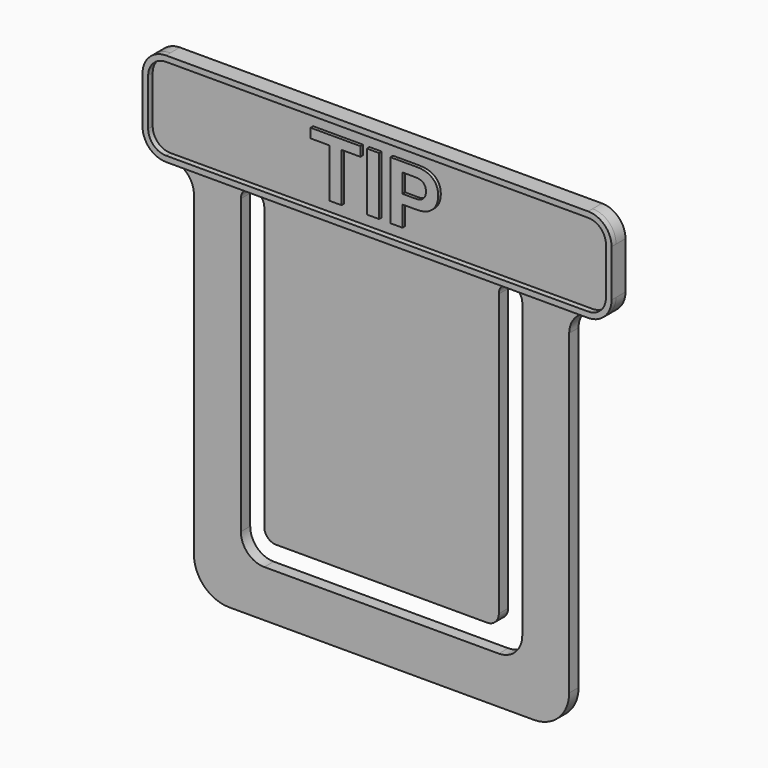
from build123d import *

# Parameters (mm, degrees)
F0_W          = 25.4
F0_H          = 25.4
F1_DEPTH      = 0.79375
F2_R          = 2.38125
F3_W          = 19.05
F3_H          = 22.225
F4_DEPTH      = 4.9276
F6_DEPTH      = 0.79375
F7_R          = 1.58749
F8_R          = 1.5875
F9_W          = 15.875
F9_H          = 20.6375
F10_DEPTH     = 0.79375
F11_R         = 0.79374
F12_R         = 0.79375
F14_DEPTH     = 0.381
F16_DEPTH     = 0.381
F17_TEXT_SIZE = 5.7207213508
F18_DEPTH     = 1.016


# Not quite as in the source:
# - a fillet or chamfer is up to 0.001 mm smaller than in the source, because OpenCascade refuses the exact size
# - ends of sketch curves that miss each other by under 0.0002 mm in the source are joined
# - Text() gives the source's letters only with a copy of the font that has no kerning and outlines rounded to 1/6400 em; it was checked with that copy


with BuildPart() as f1:
    # F0 (on Front) → F1 (new body)
    with BuildSketch(Plane.XZ):
        Rectangle(F0_W, F0_H)
    extrude(amount=F1_DEPTH)

    # F2
    f2_edges = [f1.edges().sort_by_distance(p)[0] for p in [
        (12.7, -0.396875, -12.7),
        (-12.7, -0.396875, -12.7),
    ]]
    fillet(f2_edges, radius=F2_R)

    # F3 (on face) → F4 (cut)
    with BuildSketch(Plane.XZ.offset(0.79375)):
        with Locations((0, 1.5875)):
            Rectangle(F3_W, F3_H)
    extrude(amount=-F4_DEPTH, mode=Mode.SUBTRACT)

    # F5 (on face) → F6 (join)
    with BuildSketch(Plane.XZ.offset(0.79375)):
        Polygon((-15.875, 19.05), (-15.875, 12.7), (-12.7, 12.7), (-9.525, 12.7), (9.525, 12.7), (12.7, 12.7), (15.875, 12.7), (15.875, 19.05), align=None)
    extrude(amount=-F6_DEPTH)

    # F7 (radius 1.5875 in the source; OpenCascade refuses exactly that, so slightly less here)
    f7_edges = [f1.edges().sort_by_distance(p)[0] for p in [
        (-15.875, -0.396875, 19.05),
        (15.875, -0.396875, 19.05),
        (15.875, -0.396875, 12.7),
        (12.7, -0.396875, 12.7),
        (-15.875, -0.396875, 12.7),
        (-12.7, -0.396875, 12.7),
    ]]
    fillet(f7_edges, radius=F7_R)

    # F8
    f8_edges = [f1.edges().sort_by_distance(p)[0] for p in [
        (-9.525, -0.396875, -9.525),
        (9.525, -0.396875, -9.525),
    ]]
    fillet(f8_edges, radius=F8_R)

    # F9 (on face) → F10 (join)
    with BuildSketch(Plane.XZ.offset(0.79375)):
        with BuildLine():
            ThreePointArc((-14.28751, 19.05), (-15.4100349441, 18.5850349441), (-15.875, 17.46251))
            Line((-15.875, 17.46251), (-15.875, 14.28749))
            ThreePointArc((-15.875, 14.28749), (-15.4100349441, 13.1649650559), (-14.28751, 12.7))
            ThreePointArc((-14.28751, 12.7), (-13.1649650559, 12.2350349441), (-12.7, 11.11251))
            Line((-12.7, 11.11251), (-12.7, -10.31875))
            ThreePointArc((-12.7, -10.31875), (-12.0025480227, -12.0025480227), (-10.31875, -12.7))
            Line((-10.31875, -12.7), (10.31875, -12.7))
            ThreePointArc((10.31875, -12.7), (12.0025480227, -12.0025480227), (12.7, -10.31875))
            Line((12.7, -10.31875), (12.7, 11.11251))
            ThreePointArc((12.7, 11.11251), (13.1649650559, 12.2350349441), (14.28749, 12.7))
            ThreePointArc((14.28749, 12.7), (15.4100349441, 13.1649650559), (15.875, 14.28749))
            Line((15.875, 14.28749), (15.875, 17.46251))
            ThreePointArc((15.875, 17.46251), (15.4100349441, 18.5850349441), (14.28751, 19.05))
            Line((14.28751, 19.05), (-14.28751, 19.05))
        make_face()
        with BuildLine():
            Line((-9.525, 12.7), (-7.9375, 12.7))
            Line((-7.9375, 12.7), (7.9375, 12.7))
            Line((7.9375, 12.7), (9.525, 12.7))
            Line((9.525, 12.7), (9.525, -7.9375))
            ThreePointArc((9.525, -7.9375), (9.0600320151, -9.0600320151), (7.9375, -9.525))
            Line((7.9375, -9.525), (-7.9375, -9.525))
            ThreePointArc((-7.9375, -9.525), (-9.0600320151, -9.0600320151), (-9.525, -7.9375))
            Line((-9.525, -7.9375), (-9.525, 12.7))
        make_face(mode=Mode.SUBTRACT)
        with Locations((0, 2.38125)):
            Rectangle(F9_W, F9_H)
    extrude(amount=-F10_DEPTH)

    # F11 (radius 0.79375 in the source; OpenCascade refuses exactly that, so slightly less here)
    f11_edges = [f1.edges().sort_by_distance(p)[0] for p in [
        (-7.9375, -0.396875, 12.7),
        (-9.525, -0.396875, 12.7),
        (7.9375, -0.396875, 12.7),
        (9.525, -0.396875, 12.7),
    ]]
    fillet(f11_edges, radius=F11_R)

    # F12
    f12_edges = [f1.edges().sort_by_distance(p)[0] for p in [
        (-7.9375, -0.396875, -7.9375),
        (7.9375, -0.396875, -7.9375),
    ]]
    fillet(f12_edges, radius=F12_R)

    # F13 (on face) → F14 (join)
    with BuildSketch(Plane.XZ.offset(0.79375)):
        with BuildLine():
            Line((14.2875, 19.05), (-14.2875, 19.05))
            ThreePointArc((-14.2875, 19.05), (-15.4100320151, 18.5850320151), (-15.875, 17.4625))
            Line((-15.875, 17.4625), (-15.875, 14.2875))
            ThreePointArc((-15.875, 14.2875), (-15.4100320151, 13.1649679849), (-14.2875, 12.7))
            Line((-14.2875, 12.7), (-8.73125, 12.7))
            Line((-8.73125, 12.7), (8.73125, 12.7))
            Line((8.73125, 12.7), (14.2875, 12.7))
            ThreePointArc((14.2875, 12.7), (15.4100320151, 13.1649679849), (15.875, 14.2875))
            Line((15.875, 14.2875), (15.875, 17.4625))
            ThreePointArc((15.875, 17.4625), (15.4100320151, 18.5850320151), (14.2875, 19.05))
        make_face()
    extrude(amount=F14_DEPTH)

    # F15 (on face) → F16 (cut, through all)
    with BuildSketch(Plane.XZ.offset(1.17475)):
        with BuildLine():
            Line((14.2875, 18.669), (-14.2875, 18.669))
            ThreePointArc((-14.2875, 18.669), (-15.1406243315, 18.3156243315), (-15.494, 17.4625))
            Line((-15.494, 17.4625), (-15.494, 14.2875))
            ThreePointArc((-15.494, 14.2875), (-15.1406243315, 13.4343756685), (-14.2875, 13.081))
            Line((-14.2875, 13.081), (14.2875, 13.081))
            ThreePointArc((14.2875, 13.081), (15.1406243315, 13.4343756685), (15.494, 14.2875))
            Line((15.494, 14.2875), (15.494, 17.4625))
            ThreePointArc((15.494, 17.4625), (15.1406243315, 18.3156243315), (14.2875, 18.669))
        make_face()
    extrude(amount=-F16_DEPTH, mode=Mode.SUBTRACT)

    # F17 (on Front) → F18 (join)
    with BuildSketch(Plane.XZ):
        with Locations((-4.6928301454, 13.8831362128)):
            Text('TIP', F17_TEXT_SIZE, font='Arimo', font_style=FontStyle.BOLD, text_align=(TextAlign.LEFT, TextAlign.BOTTOM))
    extrude(amount=F18_DEPTH)


solid = f1.part
